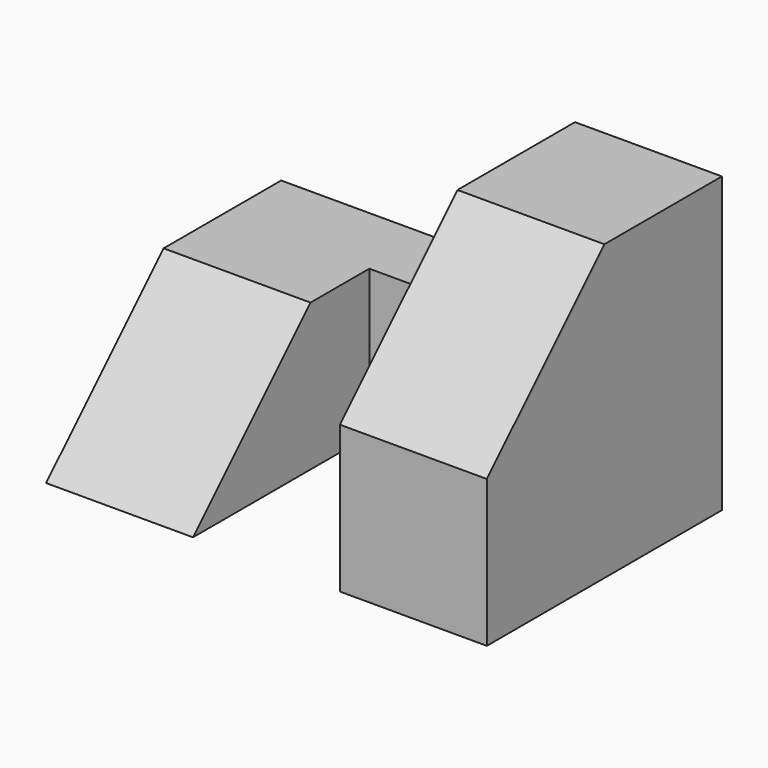
from build123d import *

# Parameters (mm, degrees)
F1_DEPTH = 12.7
F2_W     = 6.35
F2_H     = 12.7
F3_DEPTH = 12.7
F4_W     = 6.35
F4_H     = 12.7
F5_DEPTH = 12.7


with BuildPart() as f1:
    # F0 (on Right) → F1 (new body)
    with BuildSketch(Plane.YZ):
        Polygon((-25.4, 0), (0, 0), (0, 12.7), (-12.7, 12.7), align=None)
    extrude(amount=F1_DEPTH)

    # F2 (on face) → F3 (join)
    with BuildSketch(Plane.YZ.offset(12.7)):
        with Locations((-3.175, 6.35)):
            Rectangle(F2_W, F2_H)
    extrude(amount=F3_DEPTH)

    # F4 (on face) → F5 (join)
    with BuildSketch(Plane.YZ.offset(25.4)):
        with Locations((-3.175, 6.35)):
            Rectangle(F4_W, F4_H)
        Polygon((-6.35, 12.7), (0, 12.7), (0, 25.4), (-12.7, 25.4), (-25.4, 12.7), (-25.4, 0), (-6.35, 0), align=None)
    extrude(amount=F5_DEPTH)


solid = f1.part
